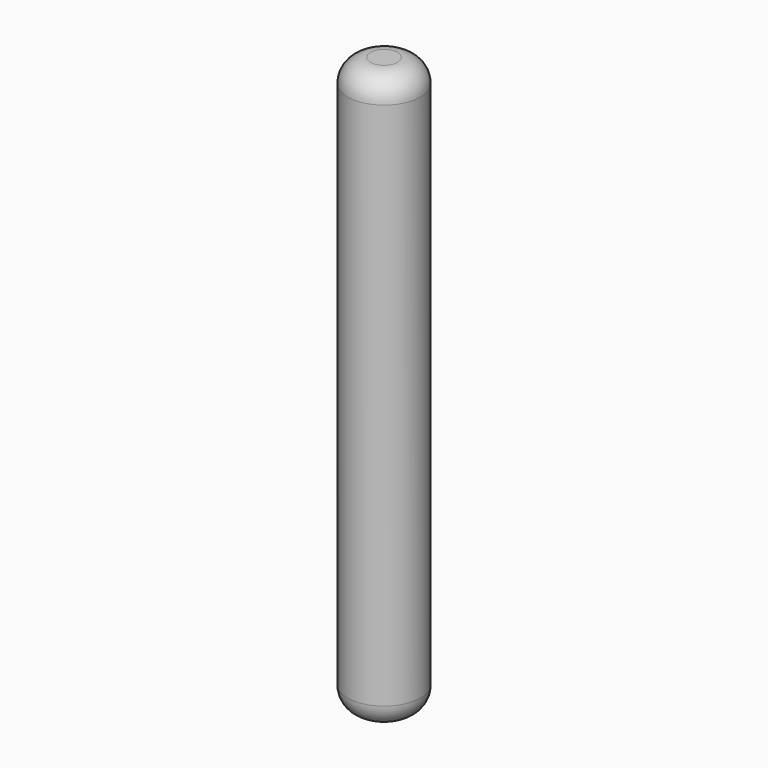
from build123d import *

# Parameters (mm, degrees)
F1_R     = 1.5875
F2_DEPTH = 25
F3_R     = 1


with BuildPart() as f2:
    # F1 (on Top) → F2 (new body)
    with BuildSketch(Plane.XY):
        Circle(F1_R)
    extrude(amount=F2_DEPTH)

    # F3
    f3_edges = [f2.edges().sort_by_distance(p)[0] for p in [
        (-1.5875, 0, 25),
        (-1.5875, 0, 0),
    ]]
    fillet(f3_edges, radius=F3_R)


solid = f2.part
